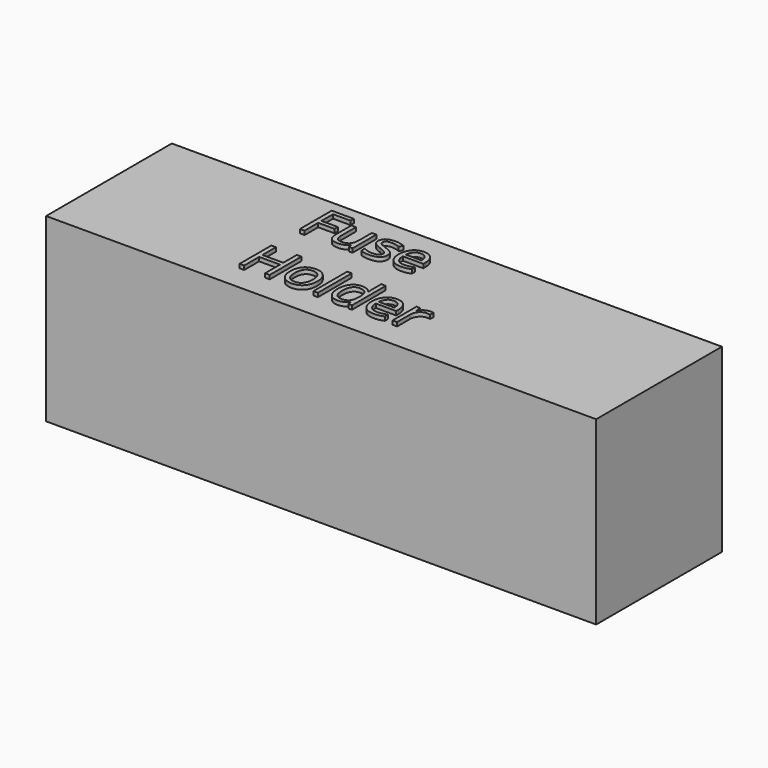
from build123d import *

# Parameters (mm, degrees)
F0_W         = 177.8
F0_H         = 50.8
F1_DEPTH     = 58.42
F2_TEXT_SIZE = 17.9489304881
F3_DEPTH     = 1.27


# Not quite as in the source:
# - Text() gives the source's letters only with a copy of the font that has no kerning and outlines rounded to 1/6400 em; it was checked with that copy


with BuildPart() as f1:
    # F0 (on Top) → F1 (new body)
    with BuildSketch(Plane.XY):
        with Locations((-11.3581030496, -2.9457365163)):
            Rectangle(F0_W, F0_H)
    extrude(amount=F1_DEPTH)

    # F2 (on face) → F3 (join)
    with BuildSketch(Plane.XY.offset(58.42)):
        with Locations((-46.0417680442, 4.2760702781)):
            Text('Fuse', F2_TEXT_SIZE, font='Open Sans', text_align=(TextAlign.LEFT, TextAlign.BOTTOM))
        with Locations((-46.0417680442, -20.1344751856)):
            Text('Holder', F2_TEXT_SIZE, font='Open Sans', text_align=(TextAlign.LEFT, TextAlign.BOTTOM))
    extrude(amount=F3_DEPTH)


solid = f1.part
